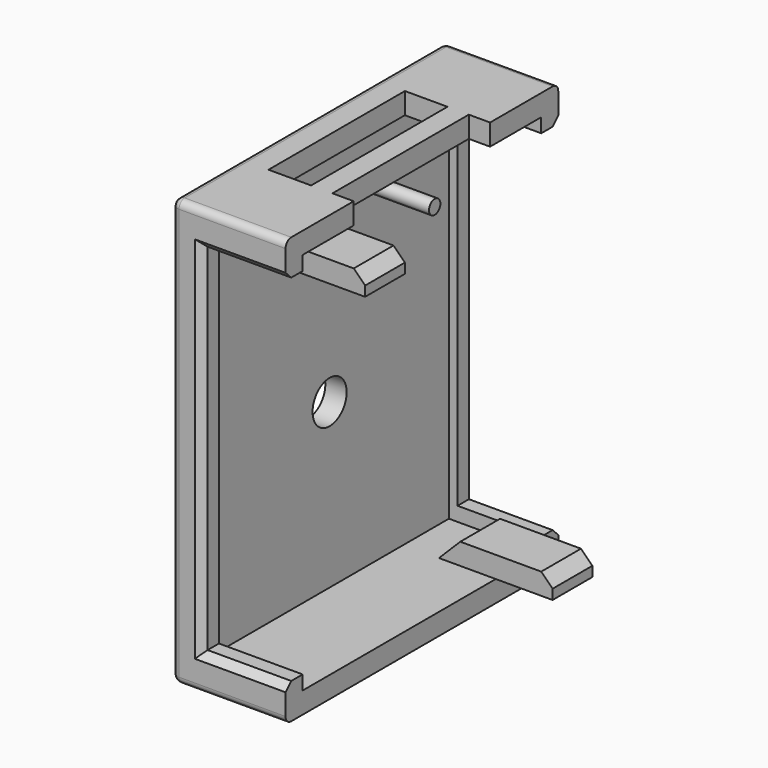
from build123d import *

# Parameters (mm, degrees)
F1_W      = 24
F1_H      = 30
F2_DEPTH  = 8
F3_T      = -1.5
F4_W      = 3
F4_H      = 12
F5_DEPTH  = 5
F6_W      = 8
F6_H      = 25
F7_DEPTH  = 30
F8_W      = 3.5
F8_H      = 1.5
F9_DEPTH  = 4
F10_SIZE  = 0.8
F11_R     = 1.5
F12_DEPTH = 25
F13_R     = 0.5
F14_SIZE  = 0.5
F15_R     = 0.5
F16_DEPTH = 5
F17_SIZE  = 1.49999


# Not quite as in the source:
# - a fillet or chamfer is up to 0.001 mm smaller than in the source, because OpenCascade refuses the exact size


with BuildPart() as f2:
    # F1 (on Right) → F2 (new body)
    with BuildSketch(Plane.YZ):
        with Locations((-10, -15)):
            Rectangle(F1_W, F1_H)
    extrude(amount=-F2_DEPTH)

    # F3
    f3_openings = [f2.faces().sort_by_distance(p)[0] for p in [
        (0, -10, -15),
    ]]
    offset(amount=F3_T, openings=f3_openings)

    # F4 (on Top) → F5 (cut)
    with BuildSketch(Plane.XY):
        with Locations((0, -10)):
            Rectangle(F4_W, F4_H)
        with Locations((-4.5, -10)):
            Rectangle(F4_W, F4_H)
    extrude(amount=-F5_DEPTH, mode=Mode.SUBTRACT)

    # F6 (on face) → F7 (cut)
    with BuildSketch(Plane.XZ.offset(22)):
        with Locations((-1.8903282698, -15)):
            Rectangle(F6_W, F6_H)
    extrude(amount=-F7_DEPTH, mode=Mode.SUBTRACT)

    # F8 (on Right) → F9 (join, symmetric)
    with BuildSketch(Plane.YZ):
        with Locations((-18.25, -2.25)):
            Rectangle(F8_W, F8_H)
        with Locations((-1.75, -27.75)):
            Rectangle(F8_W, F8_H)
    extrude(amount=F9_DEPTH, both=True)

    # F10
    f10_edges = [f2.edges().sort_by_distance(p)[0] for p in [
        (4, -18.25, -1.5),
        (4, -1.75, -27),
    ]]
    chamfer(f10_edges, length=F10_SIZE)

    # F11 (on Right) → F12 (cut)
    with BuildSketch(Plane.YZ):
        with Locations((-10, -17)):
            Circle(F11_R)
    extrude(amount=-F12_DEPTH, mode=Mode.SUBTRACT)

    # F13
    f13_edges = [f2.edges().sort_by_distance(p)[0] for p in [
        (-4, 2, 0),
        (-8, 2, -15),
        (-4, -22, 0),
        (-4, -22, -30),
        (-4, 2, -30),
        (-8, -10, 0),
        (-8, -22, -15),
        (-8, -10, -30),
    ]]
    fillet(f13_edges, radius=F13_R)

    # F14
    f14_edges = [f2.edges().sort_by_distance(p)[0] for p in [
        (-5.890328, 2, -15),
        (-2.945164, 2, -2.5),
        (-2.945164, 2, -27.5),
        (-2.945164, -22, -2.5),
        (-5.890328, -22, -15),
        (-2.945164, -22, -27.5),
    ]]
    chamfer(f14_edges, length=F14_SIZE)

    # F15 (on face) → F16 (join)
    with BuildSketch(Plane.YZ.offset(-6.5)):
        with Locations((-13, -4.5)):
            Circle(F15_R)
        with Locations((-7, -4.5)):
            Circle(F15_R)
    extrude(amount=F16_DEPTH)

    # F17 (size 1.5 in the source; OpenCascade refuses exactly that, so slightly less here)
    f17_edges = [f2.edges().sort_by_distance(p)[0] for p in [
        (-4, -18.25, -3),
        (-4, -1.75, -27),
    ]]
    chamfer(f17_edges, length=F17_SIZE)


solid = f2.part
